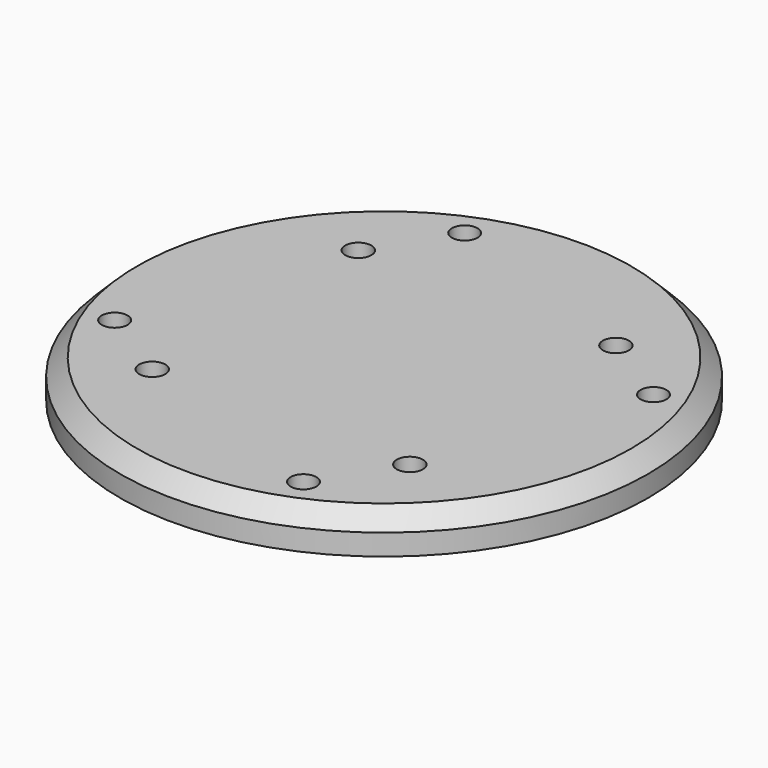
from build123d import *

# Parameters (mm, degrees)
F0_R            = 31.25
F1_DEPTH        = 4.5
F2_R            = 1.525
F3_DEPTH        = 4.501
F3_COPIES_COUNT = 4
F4_SIZE         = 2
F5_R            = 1.55
F6_DEPTH        = 4.501
F6_COPIES_COUNT = 4


# Not quite as in the source:
# - a pattern or mirror of a feature is missing from the dataset's text; its kind, count and spacing are read off the source's solid


with BuildPart() as f1:
    # F0 (on Top) → F1 (new body)
    with BuildSketch(Plane.XY):
        Circle(F0_R)
    extrude(amount=F1_DEPTH)

    # F2 (on face) → F3 (cut, through all)
    with BuildSketch(Plane.XY.offset(4.5)):
        with Locations((24.1067802187, 9.7397714288)):
            Circle(F2_R)
    f3 = extrude(amount=-F3_DEPTH, mode=Mode.SUBTRACT)

    # F3_copies: F3 ×4 about axis
    f3_copies_axis = Axis((0, 0, 0), (0, 0, 1))
    for i in range(1, F3_COPIES_COUNT):
        add(f3.rotate(f3_copies_axis, i * 360 / F3_COPIES_COUNT), mode=Mode.SUBTRACT)

    # F4
    f4_edges = [f1.edges().sort_by_distance(p)[0] for p in [
        (-31.25, 0, 4.5),
    ]]
    chamfer(f4_edges, length=F4_SIZE)

    # F5 (on face) → F6 (cut, through all)
    with BuildSketch(Plane.XY.offset(4.5)):
        with Locations((15.25, 15.25)):
            Circle(F5_R)
    f6 = extrude(amount=-F6_DEPTH, mode=Mode.SUBTRACT)

    # F6_copies: F6 ×4 about axis
    f6_copies_axis = Axis((0, 0, 0), (0, 0, 1))
    for i in range(1, F6_COPIES_COUNT):
        add(f6.rotate(f6_copies_axis, i * 360 / F6_COPIES_COUNT), mode=Mode.SUBTRACT)


solid = f1.part
